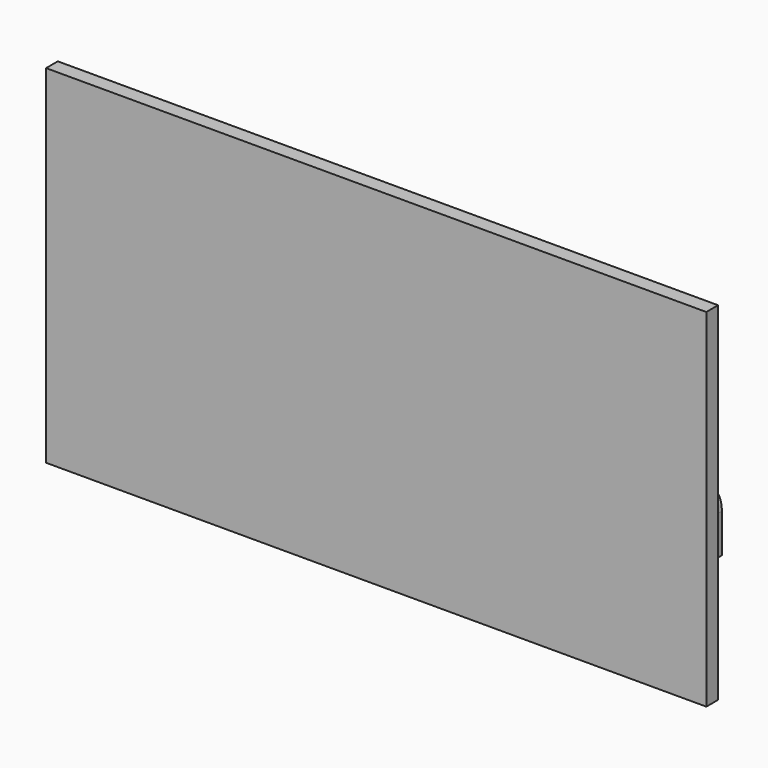
from build123d import *

# Parameters (mm, degrees)
F0_W           = 45
F0_H           = 35
F1_DEPTH       = 1
F2_TEXT_SIZE   = 8.2925846868
F2_TEXT_SIZE_2 = 7.4450868777
F2_TEXT_SIZE_3 = 6.1745380604
F3_DEPTH       = 1
F4_W           = 45
F4_H           = 11.3187799134
F5_DEPTH       = 25.4
F8_DEPTH       = 2


# Not quite as in the source:
# - Text() gives the source's letters only with a copy of the font that has no kerning and outlines rounded to 1/6400 em; it was checked with that copy


with BuildPart() as f1:
    # F0 (on Front) → F1 (new body)
    with BuildSketch(Plane.XZ):
        with Locations((16.1230944097, 8.9404625169)):
            Rectangle(F0_W, F0_H)
    extrude(amount=F1_DEPTH)

    # F2 (on face) → F3 (join)
    with BuildSketch(Plane.XZ.offset(1)):
        with Locations((-6.3769055903, 18.2020762196)):
            Text('Volvo', F2_TEXT_SIZE, font='Open Sans', font_style=FontStyle.BOLD, text_align=(TextAlign.LEFT, TextAlign.BOTTOM))
        with Locations((5.1588571388, 10.8535233609)):
            Text('Experten', F2_TEXT_SIZE_2, font='Open Sans', font_style=FontStyle.BOLD, text_align=(TextAlign.LEFT, TextAlign.BOTTOM))
        with Locations((-0.3513807805, 3.6738085225)):
            Text('Stockholm', F2_TEXT_SIZE_3, font='Open Sans', font_style=FontStyle.BOLD, text_align=(TextAlign.LEFT, TextAlign.BOTTOM))
    extrude(amount=F3_DEPTH)

    # F4 (on face) → F5 (cut)
    with BuildSketch(Plane.XZ.offset(1)):
        with Locations((16.1230944097, -2.9001475264)):
            Rectangle(F4_W, F4_H)
    extrude(amount=-F5_DEPTH, mode=Mode.SUBTRACT)


with BuildPart() as f6_1:
    # F6: instance of F1
    add(f1.part.mirror(Plane.XZ))


with BuildPart() as f1_1:
    add(f1.part)

    # F7 (on face) → F8 (cut)
    with BuildSketch(Plane.XZ.offset(2)):
        Polygon((40.6377725303, 27.0310658962), (-7.326960098, 27.0310658962), (-7.1846307255, 1.198428683), (40.6377725303, 1.198428683), align=None)
    extrude(amount=-F8_DEPTH, mode=Mode.SUBTRACT)


solid = f6_1.part
